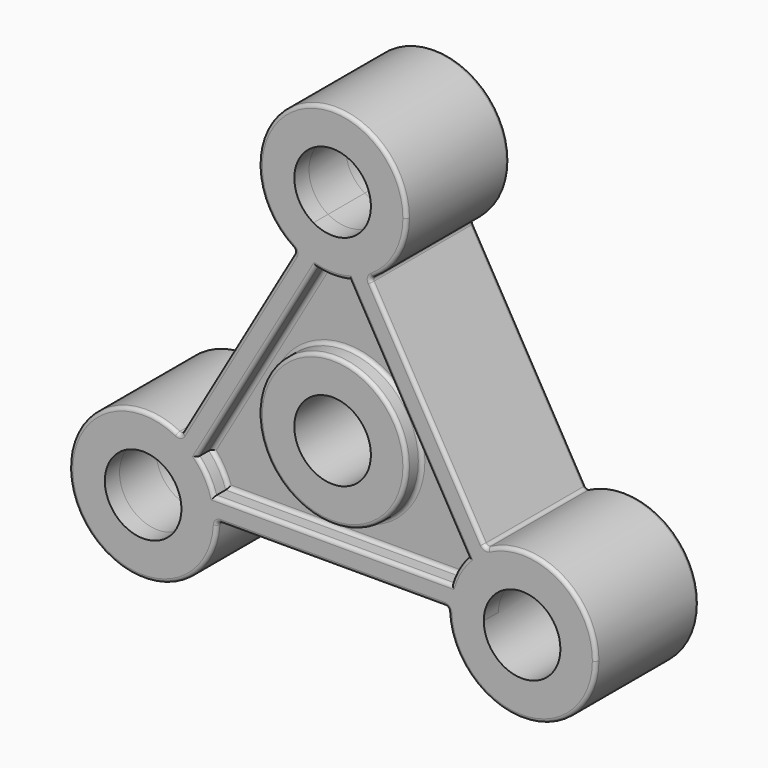
from build123d import *

# Parameters (mm, degrees)
F2_R     = 5.1196510071
F2_R_2   = 2.6515616386
F3_DEPTH = 3.175
F1_DEPTH = 4.445
F4_F1_R  = 0.254
F4_F2_R  = 0.254
F4_F3_R  = 0.2539


# Not quite as in the source:
# - a fillet or chamfer is up to 0.001 mm smaller than in the source, because OpenCascade refuses the exact size


with BuildPart() as f3:
    # F2 (on Front) → F3 (new body, symmetric)
    with BuildSketch(Plane.XZ):
        with BuildLine():
            ThreePointArc((-9.3806448858, -4.073376332), (-8.6834594607, -5.0133976571), (-8.2179698256, -6.0871886089))
            Line((-8.2179698256, -6.0871886089), (8.2179698256, -6.0871886089))
            ThreePointArc((8.2179698256, -6.0871886089), (8.6834594607, -5.0133976571), (9.3806448858, -4.073376332))
            Line((9.3806448858, -4.073376332), (1.1626750602, 10.160564941))
            ThreePointArc((1.1626750602, 10.160564941), (0, 10.0267953142), (-1.1626750602, 10.160564941))
            Line((-1.1626750602, 10.160564941), (-9.3806448858, -4.073376332))
        make_face()
        Circle(F2_R, mode=Mode.SUBTRACT)
        Circle(F2_R)
        Circle(F2_R_2, mode=Mode.SUBTRACT)
        with BuildLine():
            Line((-7.9975562842, -7.5732231607), (-10.4656456527, -7.5732231607))
            ThreePointArc((-10.4656456527, -7.5732231607), (-15.4135270301, -8.89900398), (-11.791426472, -5.2769034219))
            Line((-11.791426472, -5.2769034219), (-10.5573817878, -3.13947533))
            ThreePointArc((-10.5573817878, -3.13947533), (-17.5509551221, -10.1330486643), (-7.9975562842, -7.5732231607))
        make_face()
        with BuildLine():
            Line((10.4656456527, -7.5732231607), (7.9975562842, -7.5732231607))
            ThreePointArc((7.9975562842, -7.5732231607), (13.1172072914, -12.6928741678), (18.2368582985, -7.5732231607))
            ThreePointArc((18.2368582985, -7.5732231607), (15.6770327949, -3.13947533), (10.5573817878, -3.13947533))
            Line((10.5573817878, -3.13947533), (11.791426472, -5.2769034219))
            ThreePointArc((11.791426472, -5.2769034219), (14.4429881107, -5.2769034219), (15.76876893, -7.5732231607))
            ThreePointArc((15.76876893, -7.5732231607), (13.1172072914, -10.2247847993), (10.4656456527, -7.5732231607))
        make_face()
        with BuildLine():
            ThreePointArc((5.1196510071, 15.1464463214), (-2.5598255036, 19.5801941521), (-2.5598255036, 10.7126984907))
            Line((-2.5598255036, 10.7126984907), (-1.3257808193, 12.8501265826))
            ThreePointArc((-1.3257808193, 12.8501265826), (-1.3257808193, 17.4427660601), (2.6515616386, 15.1464463214))
            ThreePointArc((2.6515616386, 15.1464463214), (2.2963197388, 13.820665502), (1.3257808193, 12.8501265826))
            Line((1.3257808193, 12.8501265826), (2.5598255036, 10.7126984907))
            ThreePointArc((2.5598255036, 10.7126984907), (4.4337478307, 12.5866208178), (5.1196510071, 15.1464463214))
        make_face()
        with BuildLine():
            ThreePointArc((-8.2179698256, -6.0871886089), (-8.0529594469, -6.8220772331), (-7.9975562842, -7.5732231607))
            Line((-7.9975562842, -7.5732231607), (7.9975562842, -7.5732231607))
            ThreePointArc((7.9975562842, -7.5732231607), (8.0529594469, -6.8220772331), (8.2179698256, -6.0871886089))
            Line((8.2179698256, -6.0871886089), (-8.2179698256, -6.0871886089))
        make_face()
        with BuildLine():
            Line((-2.5598255036, 10.7126984907), (-10.5573817878, -3.13947533))
            ThreePointArc((-10.5573817878, -3.13947533), (-9.9345719139, -3.5630288401), (-9.3806448858, -4.073376332))
            Line((-9.3806448858, -4.073376332), (-1.1626750602, 10.160564941))
            ThreePointArc((-1.1626750602, 10.160564941), (-1.881612467, 10.3851060732), (-2.5598255036, 10.7126984907))
        make_face()
        with BuildLine():
            Line((1.1626750602, 10.160564941), (9.3806448858, -4.073376332))
            ThreePointArc((9.3806448858, -4.073376332), (9.9345719139, -3.5630288401), (10.5573817878, -3.13947533))
            Line((10.5573817878, -3.13947533), (2.5598255036, 10.7126984907))
            ThreePointArc((2.5598255036, 10.7126984907), (1.881612467, 10.3851060732), (1.1626750602, 10.160564941))
        make_face()
        with BuildLine():
            ThreePointArc((-11.791426472, -5.2769034219), (-10.8208875526, -6.2474423414), (-10.4656456527, -7.5732231607))
            Line((-10.4656456527, -7.5732231607), (-7.9975562842, -7.5732231607))
            ThreePointArc((-7.9975562842, -7.5732231607), (-8.0529594469, -6.8220772331), (-8.2179698256, -6.0871886089))
            Line((-8.2179698256, -6.0871886089), (-10.5433199459, -6.0871886089))
            Line((-10.5433199459, -6.0871886089), (-9.3806448858, -4.073376332))
            ThreePointArc((-9.3806448858, -4.073376332), (-9.9345719139, -3.5630288401), (-10.5573817878, -3.13947533))
            Line((-10.5573817878, -3.13947533), (-11.791426472, -5.2769034219))
        make_face()
        with BuildLine():
            ThreePointArc((8.2179698256, -6.0871886089), (8.0529594469, -6.8220772331), (7.9975562842, -7.5732231607))
            Line((7.9975562842, -7.5732231607), (10.4656456527, -7.5732231607))
            ThreePointArc((10.4656456527, -7.5732231607), (10.8208875526, -6.2474423414), (11.791426472, -5.2769034219))
            Line((11.791426472, -5.2769034219), (10.5573817878, -3.13947533))
            ThreePointArc((10.5573817878, -3.13947533), (9.9345719139, -3.5630288401), (9.3806448858, -4.073376332))
            Line((9.3806448858, -4.073376332), (10.5433199459, -6.0871886089))
            Line((10.5433199459, -6.0871886089), (8.2179698256, -6.0871886089))
        make_face()
        with BuildLine():
            Line((-1.3257808193, 12.8501265826), (-2.5598255036, 10.7126984907))
            ThreePointArc((-2.5598255036, 10.7126984907), (-1.881612467, 10.3851060732), (-1.1626750602, 10.160564941))
            Line((-1.1626750602, 10.160564941), (0, 12.1743772179))
            Line((0, 12.1743772179), (1.1626750602, 10.160564941))
            ThreePointArc((1.1626750602, 10.160564941), (1.881612467, 10.3851060732), (2.5598255036, 10.7126984907))
            Line((2.5598255036, 10.7126984907), (1.3257808193, 12.8501265826))
            ThreePointArc((1.3257808193, 12.8501265826), (0, 12.4948846827), (-1.3257808193, 12.8501265826))
        make_face()
        with BuildLine():
            ThreePointArc((9.3806448858, -4.073376332), (8.6834594607, -5.0133976571), (8.2179698256, -6.0871886089))
            Line((8.2179698256, -6.0871886089), (10.5433199459, -6.0871886089))
            Line((10.5433199459, -6.0871886089), (9.3806448858, -4.073376332))
        make_face()
        with BuildLine():
            Line((0, 12.1743772179), (-1.1626750602, 10.160564941))
            ThreePointArc((-1.1626750602, 10.160564941), (0, 10.0267953142), (1.1626750602, 10.160564941))
            Line((1.1626750602, 10.160564941), (0, 12.1743772179))
        make_face()
        with BuildLine():
            Line((-10.5433199459, -6.0871886089), (-8.2179698256, -6.0871886089))
            ThreePointArc((-8.2179698256, -6.0871886089), (-8.6834594607, -5.0133976571), (-9.3806448858, -4.073376332))
            Line((-9.3806448858, -4.073376332), (-10.5433199459, -6.0871886089))
        make_face()
    extrude(amount=F3_DEPTH, both=True)

    # F2 (on Front) → F1 (join, symmetric)
    with BuildSketch(Plane.XZ):
        with BuildLine():
            Line((10.4656456527, -7.5732231607), (7.9975562842, -7.5732231607))
            ThreePointArc((7.9975562842, -7.5732231607), (13.1172072914, -12.6928741678), (18.2368582985, -7.5732231607))
            ThreePointArc((18.2368582985, -7.5732231607), (15.6770327949, -3.13947533), (10.5573817878, -3.13947533))
            Line((10.5573817878, -3.13947533), (11.791426472, -5.2769034219))
            ThreePointArc((11.791426472, -5.2769034219), (14.4429881107, -5.2769034219), (15.76876893, -7.5732231607))
            ThreePointArc((15.76876893, -7.5732231607), (13.1172072914, -10.2247847993), (10.4656456527, -7.5732231607))
        make_face()
        with BuildLine():
            ThreePointArc((8.2179698256, -6.0871886089), (8.0529594469, -6.8220772331), (7.9975562842, -7.5732231607))
            Line((7.9975562842, -7.5732231607), (10.4656456527, -7.5732231607))
            ThreePointArc((10.4656456527, -7.5732231607), (10.8208875526, -6.2474423414), (11.791426472, -5.2769034219))
            Line((11.791426472, -5.2769034219), (10.5573817878, -3.13947533))
            ThreePointArc((10.5573817878, -3.13947533), (9.9345719139, -3.5630288401), (9.3806448858, -4.073376332))
            Line((9.3806448858, -4.073376332), (10.5433199459, -6.0871886089))
            Line((10.5433199459, -6.0871886089), (8.2179698256, -6.0871886089))
        make_face()
        with BuildLine():
            ThreePointArc((5.1196510071, 15.1464463214), (-2.5598255036, 19.5801941521), (-2.5598255036, 10.7126984907))
            Line((-2.5598255036, 10.7126984907), (-1.3257808193, 12.8501265826))
            ThreePointArc((-1.3257808193, 12.8501265826), (-1.3257808193, 17.4427660601), (2.6515616386, 15.1464463214))
            ThreePointArc((2.6515616386, 15.1464463214), (2.2963197388, 13.820665502), (1.3257808193, 12.8501265826))
            Line((1.3257808193, 12.8501265826), (2.5598255036, 10.7126984907))
            ThreePointArc((2.5598255036, 10.7126984907), (4.4337478307, 12.5866208178), (5.1196510071, 15.1464463214))
        make_face()
        with BuildLine():
            Line((-1.3257808193, 12.8501265826), (-2.5598255036, 10.7126984907))
            ThreePointArc((-2.5598255036, 10.7126984907), (-1.881612467, 10.3851060732), (-1.1626750602, 10.160564941))
            Line((-1.1626750602, 10.160564941), (0, 12.1743772179))
            Line((0, 12.1743772179), (1.1626750602, 10.160564941))
            ThreePointArc((1.1626750602, 10.160564941), (1.881612467, 10.3851060732), (2.5598255036, 10.7126984907))
            Line((2.5598255036, 10.7126984907), (1.3257808193, 12.8501265826))
            ThreePointArc((1.3257808193, 12.8501265826), (0, 12.4948846827), (-1.3257808193, 12.8501265826))
        make_face()
        with BuildLine():
            Line((-7.9975562842, -7.5732231607), (-10.4656456527, -7.5732231607))
            ThreePointArc((-10.4656456527, -7.5732231607), (-15.4135270301, -8.89900398), (-11.791426472, -5.2769034219))
            Line((-11.791426472, -5.2769034219), (-10.5573817878, -3.13947533))
            ThreePointArc((-10.5573817878, -3.13947533), (-17.5509551221, -10.1330486643), (-7.9975562842, -7.5732231607))
        make_face()
        with BuildLine():
            ThreePointArc((-11.791426472, -5.2769034219), (-10.8208875526, -6.2474423414), (-10.4656456527, -7.5732231607))
            Line((-10.4656456527, -7.5732231607), (-7.9975562842, -7.5732231607))
            ThreePointArc((-7.9975562842, -7.5732231607), (-8.0529594469, -6.8220772331), (-8.2179698256, -6.0871886089))
            Line((-8.2179698256, -6.0871886089), (-10.5433199459, -6.0871886089))
            Line((-10.5433199459, -6.0871886089), (-9.3806448858, -4.073376332))
            ThreePointArc((-9.3806448858, -4.073376332), (-9.9345719139, -3.5630288401), (-10.5573817878, -3.13947533))
            Line((-10.5573817878, -3.13947533), (-11.791426472, -5.2769034219))
        make_face()
        Circle(F2_R)
        Circle(F2_R_2, mode=Mode.SUBTRACT)
        with BuildLine():
            Line((-10.5433199459, -6.0871886089), (-8.2179698256, -6.0871886089))
            ThreePointArc((-8.2179698256, -6.0871886089), (-8.6834594607, -5.0133976571), (-9.3806448858, -4.073376332))
            Line((-9.3806448858, -4.073376332), (-10.5433199459, -6.0871886089))
        make_face()
        with BuildLine():
            ThreePointArc((9.3806448858, -4.073376332), (8.6834594607, -5.0133976571), (8.2179698256, -6.0871886089))
            Line((8.2179698256, -6.0871886089), (10.5433199459, -6.0871886089))
            Line((10.5433199459, -6.0871886089), (9.3806448858, -4.073376332))
        make_face()
        with BuildLine():
            Line((0, 12.1743772179), (-1.1626750602, 10.160564941))
            ThreePointArc((-1.1626750602, 10.160564941), (0, 10.0267953142), (1.1626750602, 10.160564941))
            Line((1.1626750602, 10.160564941), (0, 12.1743772179))
        make_face()
        with BuildLine():
            Line((-2.5598255036, 10.7126984907), (-10.5573817878, -3.13947533))
            ThreePointArc((-10.5573817878, -3.13947533), (-9.9345719139, -3.5630288401), (-9.3806448858, -4.073376332))
            Line((-9.3806448858, -4.073376332), (-1.1626750602, 10.160564941))
            ThreePointArc((-1.1626750602, 10.160564941), (-1.881612467, 10.3851060732), (-2.5598255036, 10.7126984907))
        make_face()
        with BuildLine():
            Line((1.1626750602, 10.160564941), (9.3806448858, -4.073376332))
            ThreePointArc((9.3806448858, -4.073376332), (9.9345719139, -3.5630288401), (10.5573817878, -3.13947533))
            Line((10.5573817878, -3.13947533), (2.5598255036, 10.7126984907))
            ThreePointArc((2.5598255036, 10.7126984907), (1.881612467, 10.3851060732), (1.1626750602, 10.160564941))
        make_face()
        with BuildLine():
            ThreePointArc((-8.2179698256, -6.0871886089), (-8.0529594469, -6.8220772331), (-7.9975562842, -7.5732231607))
            Line((-7.9975562842, -7.5732231607), (7.9975562842, -7.5732231607))
            ThreePointArc((7.9975562842, -7.5732231607), (8.0529594469, -6.8220772331), (8.2179698256, -6.0871886089))
            Line((8.2179698256, -6.0871886089), (-8.2179698256, -6.0871886089))
        make_face()
    extrude(amount=F1_DEPTH, both=True)

    # F4: fillet of radius 0.254 on 61 edges, made by hand

    # F4_f1
    f4_f1_edges = [f3.edges().sort_by_distance(p)[0] for p in [
        (5.271659973, -3.175, 3.0435943045),
        (8.6834594607, -3.175, -5.0133976571),
        (0, -3.175, -6.0871886089),
        (-8.6834594607, -3.175, -5.0133976571),
        (-5.271659973, -3.175, 3.0435943045),
        (0, -3.175, 10.0267953142),
        (-5.1196510071, -3.175, 0),
        (-10.5573817878, 0, -3.13947533),
        (-7.9975562842, 0, -7.5732231607),
        (-10.5573817878, -3.81, -3.13947533),
        (-7.9975562842, -3.81, -7.5732231607),
        (-10.5573817878, 3.81, -3.13947533),
        (-7.9975562842, 3.81, -7.5732231607),
        (-5.1196510071, 3.175, 0),
        (5.271659973, 3.175, 3.0435943045),
        (8.6834594607, 3.175, -5.0133976571),
        (0, 3.175, -6.0871886089),
        (-8.6834594607, 3.175, -5.0133976571),
        (-5.271659973, 3.175, 3.0435943045),
        (0, 3.175, 10.0267953142),
        (8.2179698256, 3.81, -6.0871886089),
        (-8.2179698256, 3.81, -6.0871886089),
        (7.9975562842, 0, -7.5732231607),
        (7.9975562842, -3.81, -7.5732231607),
        (7.9975562842, 3.81, -7.5732231607),
        (10.5573817878, 0, -3.13947533),
        (2.5598255036, 0, 10.7126984907),
        (10.5573817878, -3.81, -3.13947533),
        (2.5598255036, -3.81, 10.7126984907),
        (10.5573817878, 3.81, -3.13947533),
        (2.5598255036, 3.81, 10.7126984907),
        (-2.5598255036, 0, 10.7126984907),
        (-2.5598255036, 3.81, 10.7126984907),
        (-2.5598255036, -3.81, 10.7126984907),
    ]]
    fillet(f4_f1_edges, radius=F4_F1_R)

    # F4_f2
    f4_f2_edges = [f3.edges().sort_by_distance(p)[0] for p in [
        (-5.271659973, -4.445, 3.0435943045),
        (5.271659973, -4.445, 3.0435943045),
        (0, -4.445, 10.0267953142),
        (0, -4.445, -6.0871886089),
        (8.6834594607, -4.445, -5.0133976571),
        (-8.6834594607, -4.445, -5.0133976571),
        (-5.1196510071, -4.445, 0),
        (-5.1196510071, 4.445, 0),
        (5.271659973, 4.445, 3.0435943045),
        (-5.271659973, 4.445, 3.0435943045),
        (0, 4.445, 10.0267953142),
    ]]
    fillet(f4_f2_edges, radius=F4_F2_R)

    # F4_f3 (radius 0.254 in the source; OpenCascade refuses exactly that, so slightly less here)
    f4_f3_edges = [f3.edges().sort_by_distance(p)[0] for p in [
        (-17.5509551221, -4.445, -10.1330486643),
        (-17.5509551221, 4.445, -10.1330486643),
        (0, 4.445, 20.2660973285),
        (6.5586036457, 4.445, 3.7866115803),
        (17.5509551221, 4.445, -10.1330486643),
        (0, -4.445, 20.2660973285),
        (17.5509551221, -4.445, -10.1330486643),
        (6.5586036457, -4.445, 3.7866115803),
        (-8.729266331, 4.445, -4.9356484103),
        (0, 4.445, -6.0871886089),
        (0, -4.445, -7.5732231607),
        (0, 4.445, -7.5732231607),
        (-7.9248716183, 4.445, -7.6434222882),
        (7.9248716183, 4.445, -7.6434222882),
        (-7.9248716183, -4.445, -7.6434222882),
        (7.9248716183, -4.445, -7.6434222882),
        (8.1807654615, 4.445, -6.039836664),
        (-8.1807654615, 4.445, -6.039836664),
        (-9.4719334111, 4.445, -3.9783928764),
        (10.5818336826, -4.445, -3.041428999),
        (2.6569620643, -4.445, 10.6848512872),
        (-2.6569620643, -4.445, 10.6848512872),
        (10.5818336826, 4.445, -3.041428999),
        (2.6569620643, 4.445, 10.6848512872),
        (-2.6569620643, 4.445, 10.6848512872),
        (-10.5818336826, 4.445, -3.041428999),
        (-10.5818336826, -4.445, -3.041428999),
    ]]
    fillet(f4_f3_edges, radius=F4_F3_R)


solid = f3.part
